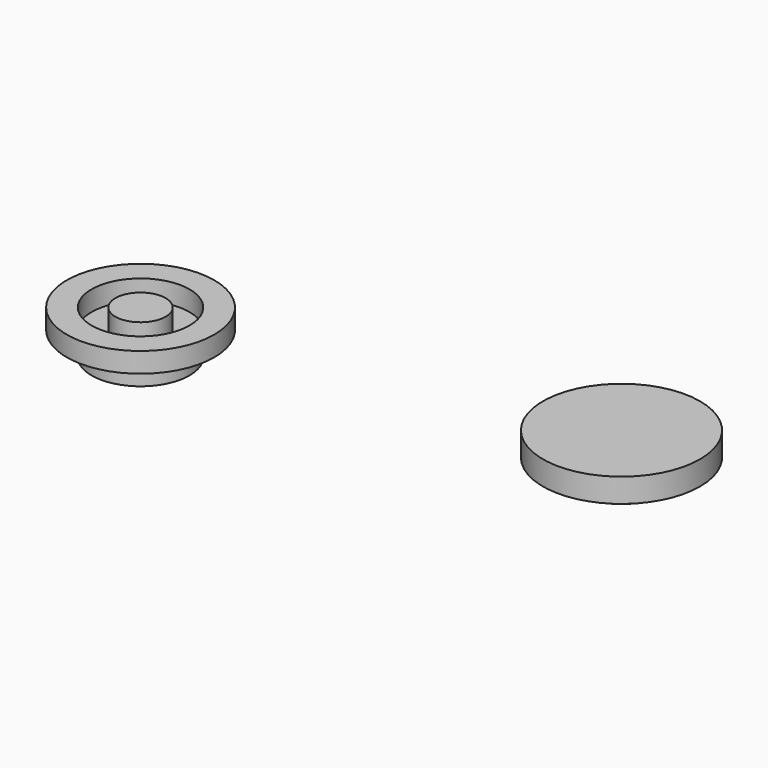
from build123d import *

# Parameters (mm, degrees)
F0_R     = 98.1955473367
F0_R_2   = 40.2352449295
F1_DEPTH = 30
F2_R     = 50.749891167
F3_DEPTH = 25
F4_R     = 61.2486550409
F4_R_2   = 31.4572402961
F5_DEPTH = 30
F6_R     = 92.1882185635
F6_R_2   = 61.2486550409
F7_DEPTH = 25
F6_R_3   = 31.4572402961


with BuildPart() as f1:
    # F0 (on Top) → F1 (new body)
    with BuildSketch(Plane.XY):
        with Locations((64.7486150265, 73.8239958882)):
            Circle(F0_R)
        with Locations((49.9009788036, 57.3229975998)):
            Circle(F0_R_2, mode=Mode.SUBTRACT)
        with Locations((49.9009788036, 57.3229975998)):
            Circle(F0_R_2)
    extrude(amount=F1_DEPTH)

    # F2 (on face) → F3 (join)
    with BuildSketch(Plane(origin=(0, 0, 0), x_dir=(1, 0, 0), z_dir=(0, 0, -1))):
        with Locations((64.7486150265, -73.8239958882)):
            Circle(F2_R)
    extrude(amount=F3_DEPTH)


with BuildPart() as f5:
    # F4 (on face) → F5 (new body)
    with BuildSketch(Plane(origin=(0, 0, -25), x_dir=(1, 0, 0), z_dir=(0, 0, -1))):
        with Locations((-499.9666213989, -28.2988809049)):
            Circle(F4_R)
        with Locations((-499.9666213989, -28.2988809049)):
            Circle(F4_R_2, mode=Mode.SUBTRACT)
    extrude(amount=F5_DEPTH)


with BuildPart() as f7:
    # F6 (on face) → F7 (new body)
    with BuildSketch(Plane.XY.offset(-25)):
        with Locations((-499.9666213989, 28.2988809049)):
            Circle(F6_R)
        with Locations((-499.9666213989, 28.2988809049)):
            Circle(F6_R_2, mode=Mode.SUBTRACT)
    extrude(amount=F7_DEPTH)


with BuildPart() as f7b:
    # F6 (on face) → F7, piece 2 (new body)
    with BuildSketch(Plane.XY.offset(-25)):
        with Locations((-499.9666213989, 28.2988809049)):
            Circle(F6_R_3)
    extrude(amount=F7_DEPTH)


solid = Compound([f1.part, f5.part, f7.part, f7b.part])
